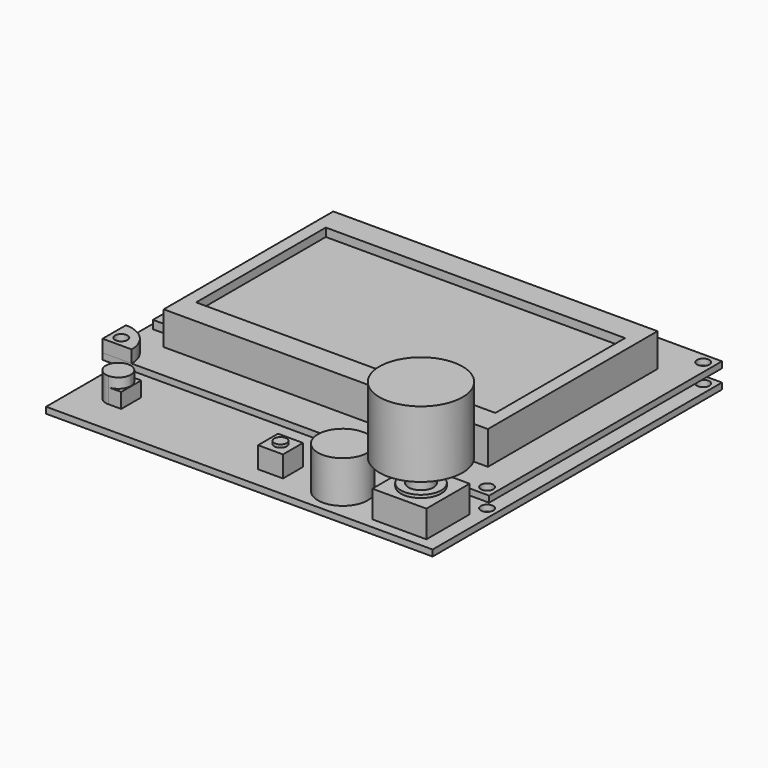
from build123d import *

# Parameters (mm, degrees)
F0_W      = 93
F0_H      = 87
F1_DEPTH  = 1.5
F3_W      = 93
F3_H      = 70
F4_DEPTH  = 1.5
F5_W      = 78
F5_H      = 51
F6_DEPTH  = 8
F7_W      = 72
F7_H      = 39
F8_DEPTH  = 2
F9_W      = 43.1
F9_H      = 2
F10_DEPTH = 6.1
F12_D     = 3
F12_2_D   = 3
F14_DEPTH = 3.6
F15_DEPTH = 6
F13_R     = 1.5
F16_DEPTH = 5.8
F13_W     = 6
F13_H     = 6
F17_DEPTH = 5.1
F13_R_2   = 6
F18_DEPTH = 10.1
F13_W_2   = 13
F13_H_2   = 13
F13_R_3   = 4.85
F13_R_4   = 3
F19_DEPTH = 6.5
F20_DEPTH = 7.2
F21_DEPTH = 26
F23_R     = 10
F24_DEPTH = 16
F25_R     = 1.5
F26_DEPTH = 3


with BuildPart() as f1:
    # F0 (on Top) → F1 (new body)
    with BuildSketch(Plane.XY):
        Rectangle(F0_W, F0_H)
    extrude(amount=F1_DEPTH)

    # F12 (through all)
    with Locations(Plane.XY.offset(6)):
        with Locations((-44, 41), (44, 41), (44, -24), (-44, -24)):
            Hole(F12_D / 2)


with BuildPart() as f4:
    # F3 (on offset) → F4 (new body)
    with BuildSketch(Plane.XY.offset(4.5)):
        with Locations((0, 8.5)):
            Rectangle(F3_W, F3_H)
    extrude(amount=F4_DEPTH)

    # F12#2 (through all)
    with Locations(Plane.XY.offset(6)):
        with Locations((-44, 41), (44, 41), (44, -24), (-44, -24)):
            Hole(F12_2_D / 2)


with BuildPart() as f6:
    # F5 (on face) → F6 (new body)
    with BuildSketch(Plane.XY.offset(6)):
        with Locations((0, 8)):
            Rectangle(F5_W, F5_H)
    extrude(amount=F6_DEPTH)

    # F7 (on face) → F8 (cut)
    with BuildSketch(Plane.XY.offset(14)):
        with Locations((0, 8)):
            Rectangle(F7_W, F7_H)
    extrude(amount=-F8_DEPTH, mode=Mode.SUBTRACT)


with BuildPart() as f10:
    # F9 (on face) → F10 (new body)
    with BuildSketch(Plane(origin=(-39, 0, 0), x_dir=(0, -1, 0), z_dir=(-1, 0, 0))):
        with Locations((-8.45, 7)):
            Rectangle(F9_W, F9_H)
    extrude(amount=F10_DEPTH)


with BuildPart() as f14:
    # F13 (on face) → F14 (new body)
    with BuildSketch(Plane.XY.offset(1.5)):
        with BuildLine():
            ThreePointArc((-38, -35.4), (-35.8786796564, -34.5213203436), (-35, -32.4))
            ThreePointArc((-35, -32.4), (-35.8786796564, -30.2786796564), (-38, -29.4))
            Line((-38, -29.4), (-38, -35.4))
        make_face()
        with BuildLine():
            ThreePointArc((-38, -29.4), (-35.8786796564, -30.2786796564), (-35, -32.4))
            ThreePointArc((-35, -32.4), (-35.8786796564, -34.5213203436), (-38, -35.4))
            Line((-38, -35.4), (-34.9, -35.4))
            Line((-34.9, -35.4), (-34.9, -29.4))
            Line((-34.9, -29.4), (-38, -29.4))
        make_face()
    extrude(amount=F14_DEPTH)

    # F13 (on face) → F15 (join)
    with BuildSketch(Plane.XY.offset(1.5)):
        with BuildLine():
            Line((-38, -35.4), (-38, -29.4))
            ThreePointArc((-38, -29.4), (-41, -32.4), (-38, -35.4))
        make_face()
        with BuildLine():
            ThreePointArc((-38, -35.4), (-35.8786796564, -34.5213203436), (-35, -32.4))
            ThreePointArc((-35, -32.4), (-35.8786796564, -30.2786796564), (-38, -29.4))
            Line((-38, -29.4), (-38, -35.4))
        make_face()
    extrude(amount=F15_DEPTH)


with BuildPart() as f16:
    # F13 (on face) → F16 (new body)
    with BuildSketch(Plane.XY.offset(1.5)):
        with Locations((3.5, -35.5)):
            Circle(F13_R)
    extrude(amount=F16_DEPTH)


with BuildPart() as f17:
    # F13 (on face) → F17 (new body)
    with BuildSketch(Plane.XY.offset(1.5)):
        with Locations((3.5, -35.5)):
            Rectangle(F13_W, F13_H)
        with Locations((3.5, -35.5)):
            Circle(F13_R, mode=Mode.SUBTRACT)
    extrude(amount=F17_DEPTH)


with BuildPart() as f18:
    # F13 (on face) → F18 (new body)
    with BuildSketch(Plane.XY.offset(1.5)):
        with Locations((18.5, -35.5)):
            Circle(F13_R_2)
    extrude(amount=F18_DEPTH)


with BuildPart() as f19:
    # F13 (on face) → F19 (new body)
    with BuildSketch(Plane.XY.offset(1.5)):
        with Locations((36.5, -34.5)):
            Rectangle(F13_W_2, F13_H_2)
        with Locations((36.5, -34.5)):
            Circle(F13_R_3, mode=Mode.SUBTRACT)
        with Locations((36.5, -34.5)):
            Circle(F13_R_3)
        with Locations((36.5, -34.5)):
            Circle(F13_R_4, mode=Mode.SUBTRACT)
        with Locations((36.5, -34.5)):
            Circle(F13_R_4)
    extrude(amount=F19_DEPTH)

    # F13 (on face) → F20 (join)
    with BuildSketch(Plane.XY.offset(1.5)):
        with Locations((36.5, -34.5)):
            Circle(F13_R_3)
        with Locations((36.5, -34.5)):
            Circle(F13_R_4, mode=Mode.SUBTRACT)
        with Locations((36.5, -34.5)):
            Circle(F13_R_4)
    extrude(amount=F20_DEPTH)

    # F13 (on face) → F21 (join)
    with BuildSketch(Plane.XY.offset(1.5)):
        with Locations((36.5, -34.5)):
            Circle(F13_R_4)
    extrude(amount=F21_DEPTH)


with BuildPart() as f24:
    # F23 (on offset) → F24 (new body)
    with BuildSketch(Plane.XY.offset(14.1)):
        with Locations((36.5, -34.5)):
            Circle(F23_R)
    extrude(amount=F24_DEPTH)


with BuildPart() as f26:
    # F25 (on face) → F26 (new body)
    with BuildSketch(Plane.XY.offset(6)):
        with BuildLine():
            Line((-46.5, -19.5), (-46.5, -26.5))
            Line((-46.5, -26.5), (-39.5, -26.5))
            ThreePointArc((-39.5, -26.5), (-41.5502525317, -21.5502525317), (-46.5, -19.5))
        make_face()
        with Locations((-44, -24)):
            Circle(F25_R, mode=Mode.SUBTRACT)
    extrude(amount=F26_DEPTH)


solid = Compound([f1.part, f4.part, f6.part, f10.part, f14.part, f16.part, f17.part, f18.part, f19.part, f24.part, f26.part])
